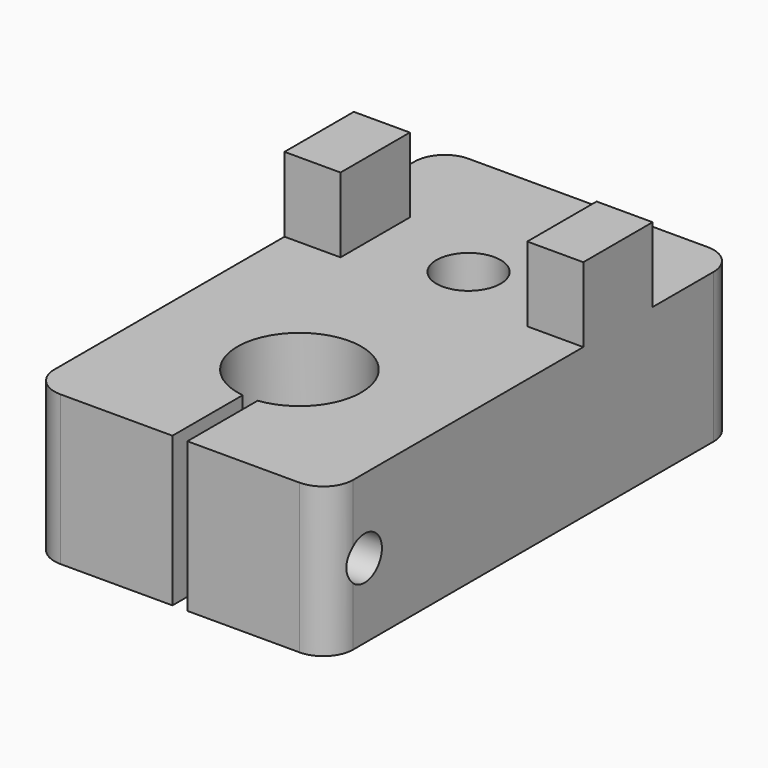
from build123d import *

# Parameters (mm, degrees)
F0_R        = 2.15
F1_DEPTH    = 10
F2_W        = 3.75
F2_H        = 5.8
F3_DEPTH    = 5
F4_R        = 1.45
F5_DEPTH    = 25
F6_T1_DEPTH = 20


# Not quite as in the source:
# - a fillet or chamfer that OpenCascade refuses, or shapes differently, is made with other operations: its cross-section is extruded or revolved along the edge and cut away or added


with BuildPart() as f1:
    # F0 (on Top) → F1 (new body)
    with BuildSketch(Plane.XY):
        with BuildLine():
            Line((-7.6355537636, 34.15), (-7.6355537636, 0))
            Line((-7.6355537636, 0), (1.8644462364, 0))
            Line((1.8644462364, 0), (1.8644462364, 2.2661458509))
            ThreePointArc((1.8644462364, 2.2661458509), (-2.9359075253, 15.6540914389), (10.1144462364, 10))
            ThreePointArc((10.1144462364, 10), (8.0185376754, 4.6996462382), (2.8644462364, 2.2661458509))
            Line((2.8644462364, 2.2661458509), (2.8644462364, 0))
            Line((2.8644462364, 0), (12.3644462364, 0))
            Line((12.3644462364, 0), (12.3644462364, 34.15))
            Line((12.3644462364, 34.15), (-7.6355537636, 34.15))
        make_face()
        with Locations((2.3644462364, 24.15)):
            Circle(F0_R, mode=Mode.SUBTRACT)
        with BuildLine():
            ThreePointArc((10.1144462364, 10), (-2.9359075253, 15.6540914389), (1.8644462364, 2.2661458509))
            Line((1.8644462364, 2.2661458509), (1.8644462364, 5.880230589))
            ThreePointArc((1.8644462364, 5.880230589), (-0.387598458, 13.1062437123), (6.5144462364, 10))
            ThreePointArc((6.5144462364, 10), (5.4706899487, 7.2479553056), (2.8644462364, 5.880230589))
            Line((2.8644462364, 5.880230589), (2.8644462364, 2.2661458509))
            ThreePointArc((2.8644462364, 2.2661458509), (8.0185376754, 4.6996462382), (10.1144462364, 10))
        make_face()
    extrude(amount=F1_DEPTH)

    # F2 (on face) → F3 (join)
    with BuildSketch(Plane.XY.offset(10)):
        with Locations((-5.7605537636, 24.15)):
            Rectangle(F2_W, F2_H)
        with Locations((10.4894462364, 24.15)):
            Rectangle(F2_W, F2_H)
    extrude(amount=F3_DEPTH)

    # F4 (on face) → F5 (cut)
    with BuildSketch(Plane.YZ.offset(12.3644462364)):
        with Locations((2.95, 5)):
            Circle(F4_R)
    extrude(amount=-F5_DEPTH, mode=Mode.SUBTRACT)

    # F6: fillet of radius 2 on 4 edges, made by hand

    # F6_s2 → F6_t1 (cut)
    with BuildSketch(Plane.XY.offset(-5)):
        with BuildLine():
            ThreePointArc((12.3644462364, 2), (11.7786597988, 0.5857864376), (10.3644462364, 0))
            Line((10.3644462364, 0), (12.3644462364, 0))
            Line((12.3644462364, 0), (12.3644462364, 2))
        make_face()
        with BuildLine():
            ThreePointArc((-7.6355537636, 2), (-7.0497673259, 0.5857864376), (-5.6355537636, 0))
            Line((-5.6355537636, 0), (-7.6355537636, 0))
            Line((-7.6355537636, 0), (-7.6355537636, 2))
        make_face()
        with BuildLine():
            ThreePointArc((10.3644462364, 34.15), (11.7786597988, 33.5642135624), (12.3644462364, 32.15))
            Line((12.3644462364, 32.15), (12.3644462364, 34.15))
            Line((12.3644462364, 34.15), (10.3644462364, 34.15))
        make_face()
        with BuildLine():
            ThreePointArc((-5.6355537636, 34.15), (-7.0497673259, 33.5642135624), (-7.6355537636, 32.15))
            Line((-7.6355537636, 32.15), (-7.6355537636, 34.15))
            Line((-7.6355537636, 34.15), (-5.6355537636, 34.15))
        make_face()
    extrude(amount=F6_T1_DEPTH, mode=Mode.SUBTRACT)


solid = f1.part
